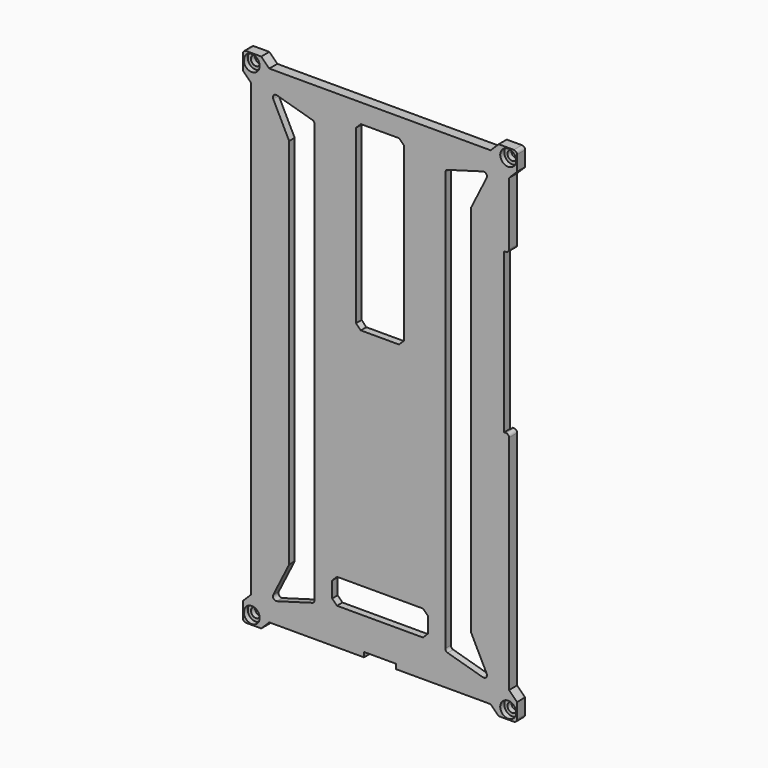
from build123d import *

# Parameters (mm, degrees)
F1_R      = 1.5
F1_W      = 24
F1_H      = 4
F2_DEPTH  = 3.175
F3_SIZE   = 2.49999
F4_R      = 1
F5_R      = 2.5
F6_DEPTH  = 1.5875
F7_W      = 15
F7_H      = 57
F7_W_2    = 30
F7_H_2    = 8
F8_DEPTH  = 3.176
F9_SIZE   = 1.5
F10_SIZE  = 1.5
F11_R     = 1
F12_W     = 78.25
F12_H     = 150.25
F13_DEPTH = 1


# Not quite as in the source:
# - a fillet or chamfer is up to 0.001 mm smaller than in the source, because OpenCascade refuses the exact size


with BuildPart() as f2:
    # F1 (on Front) → F2 (new body)
    with BuildSketch(Plane.XZ):
        Polygon((43, 73.2426406871), (43, 79), (37.2426406871, 79), (37.2426406871, 76.5), (-37.2426406871, 76.5), (-37.2426406871, 79), (-43, 79), (-43, 73.2426406871), (-40.5, 73.2426406871), (-40.5, -73.2426406871), (-43, -73.2426406871), (-43, -79), (-37.2426406871, -79), (-37.2426406871, -76.5), (-5, -76.5), (-5, -75), (5, -75), (5, -76.5), (37.2426406871, -76.5), (37.2426406871, -79), (43, -79), (43, -73.2426406871), (40.5, -73.2426406871), (40.5, 0), (39, 0), (39, 50), (40.5, 50), (40.5, 73.2426406871), align=None)
        with Locations((-40.2426406871, -76.2426406871)):
            Circle(F1_R, mode=Mode.SUBTRACT)
        with Locations((0, -61)):
            Rectangle(F1_W, F1_H, mode=Mode.SUBTRACT)
        with Locations((40.2426406871, -76.2426406871)):
            Circle(F1_R, mode=Mode.SUBTRACT)
        with Locations((-40.2426406871, 76.2426406871)):
            Circle(F1_R, mode=Mode.SUBTRACT)
        with BuildLine():
            ThreePointArc((-7.5, 58.5), (0, 66), (7.5, 58.5))
            Line((7.5, 58.5), (7.5, 25.5))
            ThreePointArc((7.5, 25.5), (0, 18), (-7.5, 25.5))
            Line((-7.5, 25.5), (-7.5, 58.5))
        make_face(mode=Mode.SUBTRACT)
        with Locations((40.2426406871, 76.2426406871)):
            Circle(F1_R, mode=Mode.SUBTRACT)
    extrude(amount=F2_DEPTH)

    # F3 (size 2.5 in the source; OpenCascade refuses exactly that, so slightly less here)
    f3_edges = [f2.edges().sort_by_distance(p)[0] for p in [
        (-37.242641, -1.5875, 76.5),
        (-40.5, -1.5875, 73.242641),
        (37.242641, -1.5875, 76.5),
        (40.5, -1.5875, 73.242641),
        (40.5, -1.5875, -73.242641),
        (37.242641, -1.5875, -76.5),
        (-37.242641, -1.5875, -76.5),
        (-40.5, -1.5875, -73.242641),
    ]]
    chamfer(f3_edges, length=F3_SIZE)

    # F4
    f4_edges = [f2.edges().sort_by_distance(p)[0] for p in [
        (43, -1.5875, 79),
        (-43, -1.5875, 79),
        (43, -1.5875, -79),
        (-43, -1.5875, -79),
        (40.5, -1.5875, 50),
        (40.5, -1.5875, 0),
    ]]
    fillet(f4_edges, radius=F4_R)

    # F5 (on face) → F6 (cut)
    with BuildSketch(Plane.XZ.offset(3.175)):
        with Locations((-40.2426406871, 76.2426406871)):
            Circle(F5_R)
        with Locations((40.2426406871, 76.2426406871)):
            Circle(F5_R)
        with Locations((40.2426406871, -76.2426406871)):
            Circle(F5_R)
        with Locations((-40.2426406871, -76.2426406871)):
            Circle(F5_R)
    extrude(amount=-F6_DEPTH, mode=Mode.SUBTRACT)

    # F7 (on face) → F8 (cut, through all)
    with BuildSketch(Plane.XZ.offset(3.175)):
        Polygon((-20.5, -66.5), (-20.5, 66.5), (-34.5, 70.5), (-28.5, 58.5), (-28.5, -58.5), (-34.5, -70.5), align=None)
        Polygon((34.5, 70.5), (20.5, 66.5), (20.5, -66.5), (34.5, -70.5), (28.5, -58.5), (28.5, 58.5), align=None)
        with Locations((0, 42)):
            Rectangle(F7_W, F7_H)
        with Locations((0, -61)):
            Rectangle(F7_W_2, F7_H_2)
    extrude(amount=-F8_DEPTH, mode=Mode.SUBTRACT)

    # F9
    f9_edges = [f2.edges().sort_by_distance(p)[0] for p in [
        (7.5, -1.5875, 70.5),
        (-7.5, -1.5875, 70.5),
        (-7.5, -1.5875, 13.5),
        (7.5, -1.5875, 13.5),
    ]]
    chamfer(f9_edges, length=F9_SIZE)

    # F10
    f10_edges = [f2.edges().sort_by_distance(p)[0] for p in [
        (-15, -1.5875, -65),
        (-15, -1.5875, -57),
        (15, -1.5875, -57),
        (15, -1.5875, -65),
    ]]
    chamfer(f10_edges, length=F10_SIZE)

    # F11
    f11_edges = [f2.edges().sort_by_distance(p)[0] for p in [
        (-34.5, -1.5875, 70.5),
        (-20.5, -1.5875, 66.5),
        (20.5, -1.5875, 66.5),
        (34.5, -1.5875, 70.5),
        (34.5, -1.5875, -70.5),
        (20.5, -1.5875, -66.5),
        (-34.5, -1.5875, -70.5),
        (-20.5, -1.5875, -66.5),
    ]]
    fillet(f11_edges, radius=F11_R)

    # F12 (on face) → F13 (cut)
    with BuildSketch(Plane(origin=(0, 0, 0), x_dir=(-1, 0, 0), z_dir=(0, 1, 0))):
        Rectangle(F12_W, F12_H)
    extrude(amount=-F13_DEPTH, mode=Mode.SUBTRACT)


solid = f2.part
